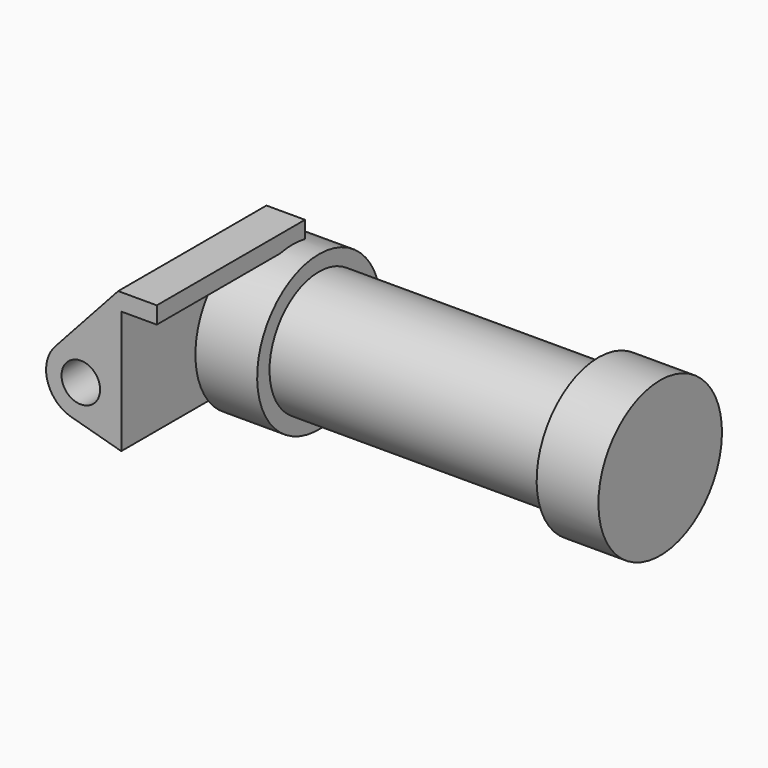
from build123d import *

# Parameters (mm, degrees)
F0_W     = 5.842
F0_H     = 12.7
F0_R     = 3.175
F2_DEPTH = 2.54
F3_DEPTH = 2.54
F4_DEPTH = 25.4


with BuildPart() as f1:
    # F0 (on Front) → F1 (revolve)
    with BuildSketch(Plane.XZ):
        with Locations((2.921, 6.35)):
            Rectangle(F0_W, F0_H)
        Polygon((5.842, 12.7), (5.842, 0), (66.294, 0), (66.294, 12.7), (56.134, 12.7), (56.134, 10.16), (10.16, 10.16), (10.16, 12.7), align=None)
    revolve(axis=Axis((33.147, 0, 0), (-1, 0, 0)))

    # F0 (on Front) → F2 (join, symmetric)
    with BuildSketch(Plane.XZ):
        with BuildLine():
            Line((5.842, 0), (0, 0))
            Line((0, 0), (-0.9398, 0))
            ThreePointArc((-0.9398, 0), (-3.195791, -4.549339), (-8.182663, -5.506983))
            Line((-8.182663, -5.506983), (5.842, -9.398))
            Line((5.842, -9.398), (5.842, 0))
        make_face()
        with BuildLine():
            ThreePointArc((-8.182663, -5.506983), (-3.195791, -4.549339), (-0.9398, 0))
            ThreePointArc((-0.9398, 0), (-4.591961, 5.329721), (-10.88063, 3.847543))
            ThreePointArc((-10.88063, 3.847543), (-12.145978, -1.583727), (-8.182663, -5.506983))
        make_face()
        with Locations((-6.6548, 0)):
            Circle(F0_R, mode=Mode.SUBTRACT)
    extrude(amount=F2_DEPTH, both=True)

    # F0 (on Front) → F3 (join, symmetric)
    with BuildSketch(Plane.XZ):
        with BuildLine():
            Line((-0.9398, 0), (0, 0))
            Line((0, 0), (0, 12.7))
            Line((0, 12.7), (5.842, 12.7))
            Line((5.842, 12.7), (5.842, 15.24))
            Line((5.842, 15.24), (-0.508, 15.24))
            Line((-0.508, 15.24), (-10.88063, 3.847543))
            ThreePointArc((-10.88063, 3.847543), (-4.591961, 5.329721), (-0.9398, 0))
        make_face()
        with Locations((2.921, 6.35)):
            Rectangle(F0_W, F0_H)
    extrude(amount=F3_DEPTH, both=True)

    # F4 (add): a face of the model
    f4_faces = [f1.faces().sort_by_distance(p)[0] for p in [
        (-3.7722, -2.54, 3.594733),
    ]]
    extrude(f4_faces, amount=F4_DEPTH)


solid = f1.part
